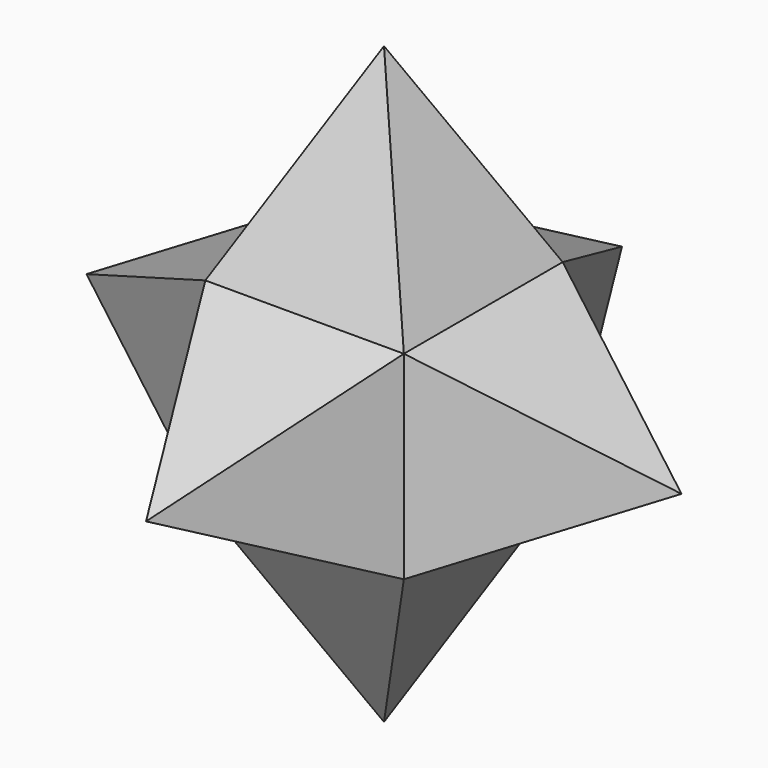
from build123d import *

# Parameters (mm, degrees)
F0_W     = 50
F0_H     = 50
F1_DEPTH = 25
F2_W     = 50
F2_H     = 50
F3_DEPTH = 50
F3_TAPER = 26.6


with BuildPart() as f1:
    # F0 (on Top) → F1 (new body, symmetric)
    with BuildSketch(Plane.XY):
        Rectangle(F0_W, F0_H)
    extrude(amount=F1_DEPTH, both=True)



with BuildPart() as f3:
    # F2 (on face) → F3 (new body)
    with BuildSketch(Plane.XY.offset(25)):
        Rectangle(F2_W, F2_H)
    extrude(amount=F3_DEPTH, taper=F3_TAPER)


with BuildPart() as f4_1:
    # F4: instance of F3
    add(f3.part.mirror(Plane.XY))


with BuildPart() as f6_1:
    # F6: instance of F3
    add(f3.part.mirror(Plane(origin=(25, -25, 25), x_dir=(-0.5773502692, 0.5773502692, -0.5773502692), z_dir=(0.7071067812, 0, -0.7071067812))))


with BuildPart() as f7_1:
    # F7: instance of F4_1
    add(f4_1.part.mirror(Plane(origin=(25, -25, 25), x_dir=(-0.5773502692, 0.5773502692, -0.5773502692), z_dir=(0.7071067812, 0, -0.7071067812))))


with BuildPart() as f9_1:
    # F9: instance of F6_1
    add(f6_1.part.mirror(Plane(origin=(25, 25, 25), x_dir=(-0.5773502692, -0.5773502692, -0.5773502692), z_dir=(0.7071067812, -0.7071067812, 0))))


with BuildPart() as f1_1:
    add(f1.part)

    add(f7_1.part)  # F10 merges F7_1
    # F10: F7_1 across plane
    add(f7_1.part.mirror(Plane(origin=(25, 25, 25), x_dir=(-0.5773502692, -0.5773502692, -0.5773502692), z_dir=(0.7071067812, -0.7071067812, 0))))


solid = Compound([f3.part, f4_1.part, f6_1.part, f9_1.part, f1_1.part])
